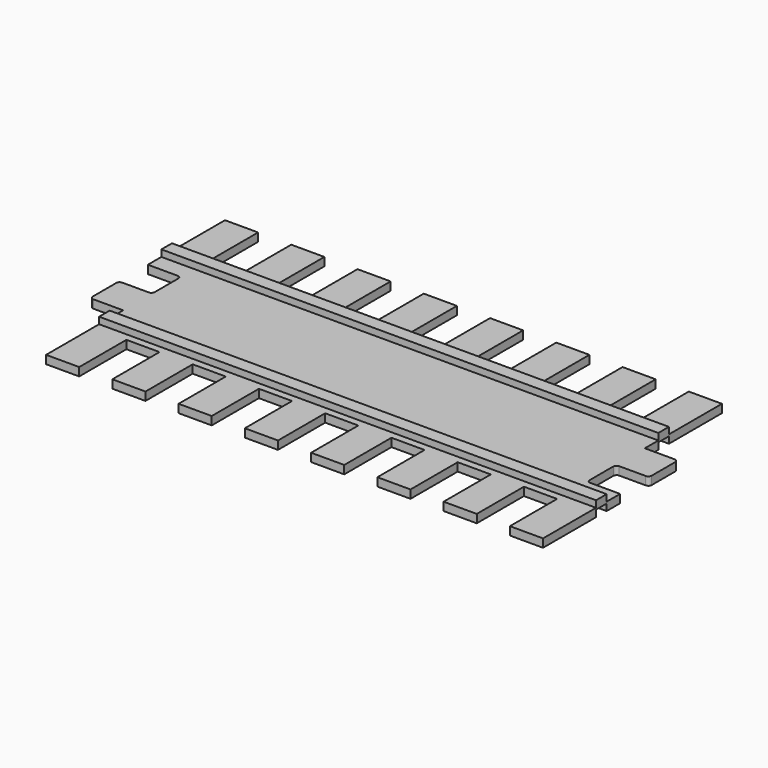
from build123d import *

# Parameters (mm, degrees)
F1_DEPTH = 3.175
F2_DEPTH = 5.715
F3_DEPTH = 2.54


# Not quite as in the source:
# - ends of sketch curves that miss each other by under 0.0002 mm in the source are joined


with BuildPart() as f1:
    # F0 (on Top) → F1 (new body)
    with BuildSketch(Plane.XY):
        Polygon((-15.470907706, -22.2827270627), (-28.170907706, -22.2827270627), (-28.170907706, -25.0712689012), (-28.170907706, -47.6827270627), (-15.470907706, -47.6827270627), (-15.470907706, -25.0712689012), (-2.770907706, -25.0712689012), (-2.770907706, -47.6827270627), (9.929092294, -47.6827270627), (9.929092294, -25.0712689012), (22.629092294, -25.0712689012), (22.629092294, -47.6827270627), (35.329092294, -47.6827270627), (35.329092294, -25.0712689012), (48.029092294, -25.0712689012), (48.029092294, -47.6827270627), (60.7290890396, -47.6827270627), (60.7290890396, -25.0712689012), (73.429092294, -25.0712689012), (73.429092294, -47.6827270627), (86.129092294, -47.6827270627), (86.129092294, -25.0712689012), (98.829092294, -25.0712689012), (98.829092294, -47.6827270627), (111.529092294, -47.6827270627), (111.529092294, -25.0712689012), (124.229092294, -25.0712689012), (124.229092294, -47.6827270627), (136.929092294, -47.6827270627), (136.929092294, -25.0712689012), (149.629092294, -25.0712689012), (149.629092294, -47.6827270627), (162.329092294, -47.6827270627), (162.329092294, -22.2827270627), (149.629092294, -22.2827270627), (136.929092294, -22.2827270627), (124.229092294, -22.2827270627), (111.529092294, -22.2827270627), (98.829092294, -22.2827270627), (86.129092294, -22.2827270627), (73.429092294, -22.2827270627), (60.729092294, -22.2827270627), (48.029092294, -22.2827270627), (35.329092294, -22.2827270627), (22.629092294, -22.2827270627), (9.929092294, -22.2827270627), (-2.770907706, -22.2827270627), align=None)
    extrude(amount=F1_DEPTH)


with BuildPart() as f1b:
    # F0 (on Top) → F1, piece 2 (new body)
    with BuildSketch(Plane.XY):
        Polygon((-40.870907706, 31.0572729373), (-40.870907706, 28.5172729373), (-28.170907706, 28.5172729373), (-15.470907706, 28.5172729373), (-2.770907706, 28.5172729373), (9.929092294, 28.5172729373), (22.629092294, 28.5172729373), (35.329092294, 28.5172729373), (48.029092294, 28.5172729373), (60.729092294, 28.5172729373), (73.429092294, 28.5172729373), (86.129092294, 28.5172729373), (98.829092294, 28.5172729373), (111.529092294, 28.5172729373), (124.229092294, 28.5172729373), (136.929092294, 28.5172729373), (149.629092294, 28.5172729373), (149.629092294, 31.0572729373), (149.629092294, 53.9172729373), (136.929092294, 53.9172729373), (136.929092294, 31.0572729373), (124.229092294, 31.0572729373), (124.229092294, 53.9172729373), (111.529092294, 53.9172729373), (111.529092294, 31.0572729373), (98.829092294, 31.0572729373), (98.829092294, 53.9172729373), (86.129092294, 53.9172729373), (86.129092294, 31.0572729373), (73.429092294, 31.0572729373), (73.429092294, 53.9172729373), (60.729092294, 53.9172729373), (60.729092294, 31.0572729373), (48.029092294, 31.0572729373), (48.029092294, 53.9172729373), (35.329092294, 53.9172729373), (35.329092294, 31.0572729373), (22.629092294, 31.0572729373), (22.629092294, 53.9172729373), (9.929092294, 53.9172729373), (9.929092294, 31.0572729373), (-2.770907706, 31.0572729373), (-2.770907706, 53.9172729373), (-15.470907706, 53.9172729373), (-15.470907706, 31.0572729373), (-28.170907706, 31.0572729373), (-28.170907706, 53.9172729373), (-40.870907706, 53.9172729373), align=None)
    extrude(amount=F1_DEPTH)


with BuildPart() as f1c:
    # F0 (on Top) → F1, piece 3 (new body)
    with BuildSketch(Plane.XY):
        with BuildLine():
            Line((149.629092294, 23.4372729373), (-40.8709011972, 23.4372729373))
            Line((-40.8709011972, 23.4372729373), (-40.870907706, 16.9602729373))
            Line((-40.870907706, 16.9602729373), (-29.440907706, 16.9602729373))
            ThreePointArc((-29.440907706, 16.9602729373), (-28.5428820939, 16.5882985494), (-28.170907706, 15.6902729373))
            Line((-28.170907706, 15.6902729373), (-28.170907706, 4.3872729373))
            ThreePointArc((-28.170907706, 4.3872729373), (-28.5428820939, 3.4892473252), (-29.440907706, 3.1172729373))
            Line((-29.440907706, 3.1172729373), (-39.600907706, 3.1172729373))
            ThreePointArc((-39.600907706, 3.1172729373), (-40.4989333181, 2.7452985494), (-40.870907706, 1.8472729373))
            Line((-40.870907706, 1.8472729373), (-40.870907706, -9.4672727573))
            ThreePointArc((-40.870907706, -9.4672727573), (-40.4989333181, -10.3652983694), (-39.600907706, -10.7372727573))
            Line((-39.600907706, -10.7372727573), (-28.170907706, -10.7372727573))
            Line((-28.170907706, -10.7372727573), (-28.170907706, -17.2027270627))
            Line((-28.170907706, -17.2027270627), (162.3290857852, -17.2027270627))
            Line((162.3290857852, -17.2027270627), (162.329092294, -10.7372727573))
            Line((162.329092294, -10.7372727573), (150.899092294, -10.7372727573))
            ThreePointArc((150.899092294, -10.7372727573), (150.0010666819, -10.3652983694), (149.629092294, -9.4672727573))
            Line((149.629092294, -9.4672727573), (149.629092294, 1.8472729373))
            ThreePointArc((149.629092294, 1.8472729373), (150.0010666819, 2.7452985494), (150.899092294, 3.1172729373))
            Line((150.899092294, 3.1172729373), (161.059092294, 3.1172729373))
            ThreePointArc((161.059092294, 3.1172729373), (161.9571179061, 3.4892473252), (162.329092294, 4.3872729373))
            Line((162.329092294, 4.3872729373), (162.329092294, 15.7018186319))
            ThreePointArc((162.329092294, 15.7018186319), (161.9571179061, 16.599844244), (161.059092294, 16.9718186319))
            Line((161.059092294, 16.9718186319), (149.629092294, 16.9718186319))
            Line((149.629092294, 16.9718186319), (149.629092294, 23.4372729373))
        make_face()
    extrude(amount=F1_DEPTH)


with BuildPart() as f2:
    # F0 (on Top) → F2 (new body)
    with BuildSketch(Plane.XY):
        Polygon((-28.170907706, 28.5172729373), (-40.870907706, 28.5172729373), (-40.870907706, 23.4372729373), (149.629092294, 23.4372729373), (149.629092294, 28.5172729373), (136.929092294, 28.5172729373), (124.229092294, 28.5172729373), (111.529092294, 28.5172729373), (98.829092294, 28.5172729373), (86.129092294, 28.5172729373), (73.429092294, 28.5172729373), (60.729092294, 28.5172729373), (48.029092294, 28.5172729373), (35.329092294, 28.5172729373), (22.629092294, 28.5172729373), (9.929092294, 28.5172729373), (-2.770907706, 28.5172729373), (-15.470907706, 28.5172729373), align=None)
    extrude(amount=F2_DEPTH)


with BuildPart() as f2b:
    # F0 (on Top) → F2, piece 2 (new body)
    with BuildSketch(Plane.XY):
        Polygon((162.3290857852, -17.2027270627), (-28.170907706, -17.2027270627), (-28.170907706, -22.2827270627), (-15.470907706, -22.2827270627), (-2.770907706, -22.2827270627), (9.929092294, -22.2827270627), (22.629092294, -22.2827270627), (35.329092294, -22.2827270627), (48.029092294, -22.2827270627), (60.729092294, -22.2827270627), (73.429092294, -22.2827270627), (86.129092294, -22.2827270627), (98.829092294, -22.2827270627), (111.529092294, -22.2827270627), (124.229092294, -22.2827270627), (136.929092294, -22.2827270627), (149.629092294, -22.2827270627), (162.329092294, -22.2827270627), align=None)
    extrude(amount=F2_DEPTH)


with BuildPart() as f3_tool:
    # F0 (on Top) → F3 (new body)
    with BuildSketch(Plane.XY):
        Polygon((-28.170907706, 28.5172729373), (-40.870907706, 28.5172729373), (-40.870907706, 23.4372729373), (149.629092294, 23.4372729373), (149.629092294, 28.5172729373), (136.929092294, 28.5172729373), (124.229092294, 28.5172729373), (111.529092294, 28.5172729373), (98.829092294, 28.5172729373), (86.129092294, 28.5172729373), (73.429092294, 28.5172729373), (60.729092294, 28.5172729373), (48.029092294, 28.5172729373), (35.329092294, 28.5172729373), (22.629092294, 28.5172729373), (9.929092294, 28.5172729373), (-2.770907706, 28.5172729373), (-15.470907706, 28.5172729373), align=None)
        Polygon((162.3290857852, -17.2027270627), (-28.170907706, -17.2027270627), (-28.170907706, -22.2827270627), (-15.470907706, -22.2827270627), (-2.770907706, -22.2827270627), (9.929092294, -22.2827270627), (22.629092294, -22.2827270627), (35.329092294, -22.2827270627), (48.029092294, -22.2827270627), (60.729092294, -22.2827270627), (73.429092294, -22.2827270627), (86.129092294, -22.2827270627), (98.829092294, -22.2827270627), (111.529092294, -22.2827270627), (124.229092294, -22.2827270627), (136.929092294, -22.2827270627), (149.629092294, -22.2827270627), (162.329092294, -22.2827270627), align=None)
    extrude(amount=F3_DEPTH)


with BuildPart() as f2_1:
    add(f2.part)

    # F3: cut by f3_tool
    add(f3_tool.part, mode=Mode.SUBTRACT)


with BuildPart() as f2b_1:
    add(f2b.part)

    # F3: cut by f3_tool
    add(f3_tool.part, mode=Mode.SUBTRACT)


solid = Compound([f1.part, f1b.part, f1c.part, f2_1.part, f2b_1.part])
